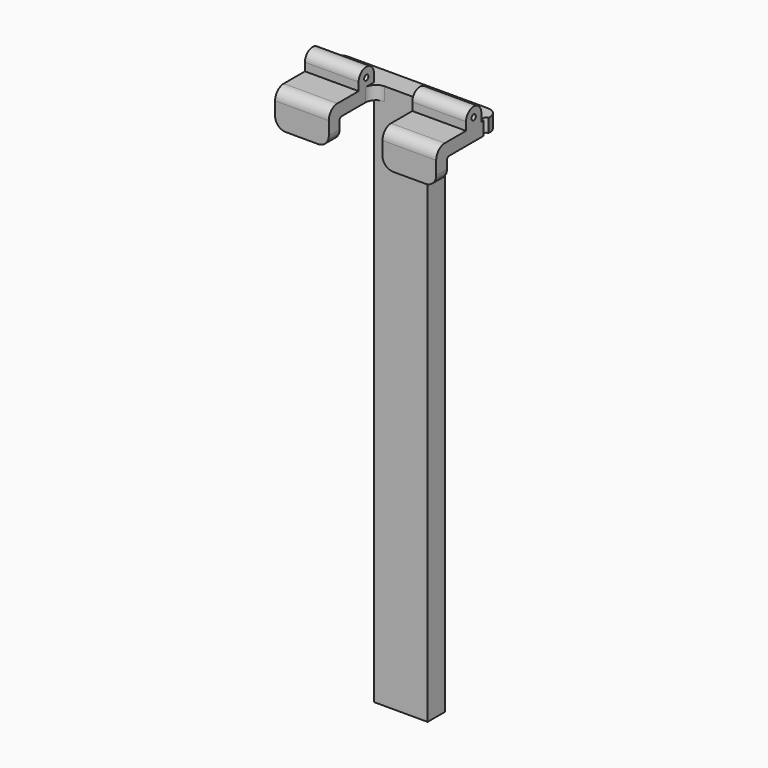
from build123d import *

# Parameters (mm, degrees)
F0_W     = 5
F0_H     = 4
F1_DEPTH = 101.6
F2_R     = 0.5
F3_DEPTH = 10
F4_R     = 2
F5_R     = 0.5
F7_DEPTH = 101.601


with BuildPart() as f1:
    # F0 (on Top) → F1 (new body)
    with BuildSketch(Plane.XY):
        with Locations((2.5, -2)):
            Rectangle(F0_W, F0_H)
    extrude(amount=-F1_DEPTH)

    # F2 (on face) → F3 (join)
    with BuildSketch(Plane.YZ.offset(5)):
        with BuildLine():
            Line((0, -2.5), (0, 0))
            Line((0, 0), (-4, 0))
            Line((-4, 0), (-4, 1.5))
            ThreePointArc((-4, 1.5), (-5.7784285378, 3.2784285378), (-7.5568570755, 1.5))
            Line((-7.5568570755, 1.5), (-7.5568570755, 0))
            Line((-7.5568570755, 0), (-14.5, 0))
            Line((-14.5, 0), (-14.5, -6.5))
            Line((-14.5, -6.5), (-12, -6.5))
            Line((-12, -6.5), (-12, -2.5))
            Line((-12, -2.5), (0, -2.5))
        make_face()
        with Locations((-5.7784285378, 1.5)):
            Circle(F2_R, mode=Mode.SUBTRACT)
    extrude(amount=F3_DEPTH)

    # F4
    f4_edges = [f1.edges().sort_by_distance(p)[0] for p in [
        (10, -14.5, 0),
        (5, -4, -1.25),
        (15, 0, -1.25),
        (15, -13.25, -6.5),
        (5, -13.25, -6.5),
    ]]
    fillet(f4_edges, radius=F4_R)

    # F5
    f5_edges = [f1.edges().sort_by_distance(p)[0] for p in [
        (10, -12, -2.5),
    ]]
    fillet(f5_edges, radius=F5_R)

    # F6 (on face) → F7 (cut, through all)
    with BuildSketch(Plane.XY):
        with BuildLine():
            Line((15, -3.4615779296), (15, -2.3238305002))
            ThreePointArc((15, -2.3238305002), (14.4311262853, -2.8927042149), (15, -3.4615779296))
        make_face()
    extrude(amount=-F7_DEPTH, mode=Mode.SUBTRACT)

    # F8: F1 across plane


with BuildPart() as f1_1:
    add(f1.part)
    add(f1.part.mirror(Plane.YZ))


solid = f1_1.part
